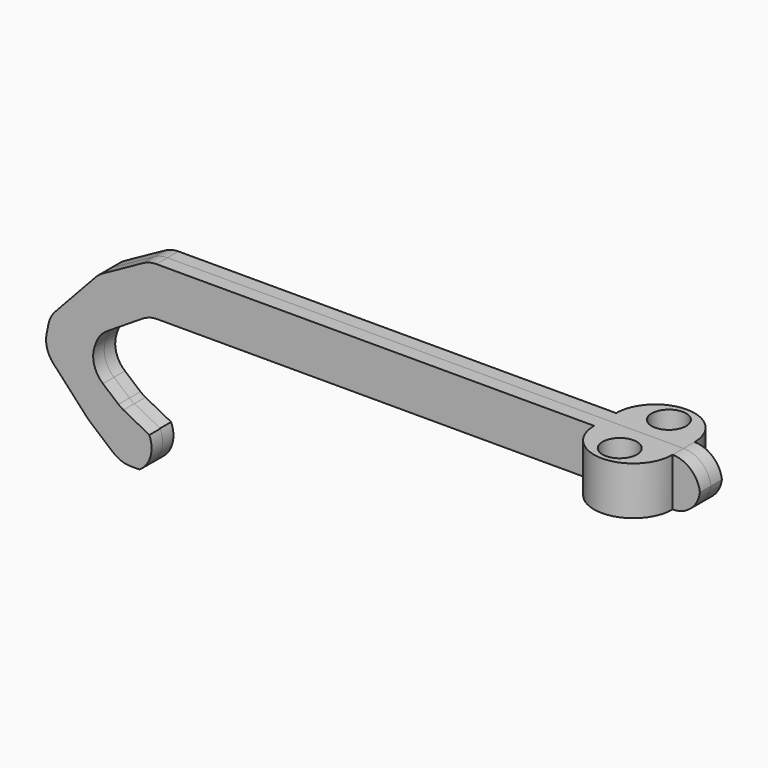
from build123d import *

# Parameters (mm, degrees)
F1_DEPTH      = 2.54
F2_T1_DEPTH   = 2.54
F2_T3_DEPTH   = 27.94
F2_T5_DEPTH   = 9.0828624111
F2_T7_DEPTH   = 6.6115491723
F2_T9_DEPTH   = 9.6489143737
F2_T11_DEPTH  = 15.5954084718
F2_T13_DEPTH  = 4.1000627259
F2_T15_DEPTH  = 11.8324981012
F4_DEPTH      = 8.89
F5_R          = 3.175
F6_DEPTH      = 25.4
F8_T1_DEPTH   = 27.7469499795
F8_2_T1_DEPTH = 27.8579477964


# Not quite as in the source:
# - a fillet or chamfer that OpenCascade refuses, or shapes differently, is made with other operations: its cross-section is extruded or revolved along the edge and cut away or added


with BuildPart() as f1:
    # F0 (on Front) → F1 (new body)
    with BuildSketch(Plane.XZ):
        Polygon((66.8724340558, 14.3756293181), (66.8724340558, 23.2656293181), (-34.7275659442, 23.2656293181), (-44.0710447729, 18.1098952889), (-53.0527345836, 8.4431990981), (-54.2040504515, 2.8466905933), (-45.9056608379, -6.1207453094), (-40.0034040213, -11.1067253005), (-36.5135949825, -11.1067253005), (-32.4798657579, -8.7494706538), (-34.7275659442, -4.9032107927), (-40.0034040213, -2.1392893977), (-45.9056608379, 2.8466905933), (-44.0710447729, 8.4431990981), (-34.7275659442, 14.3756293181), align=None)
    extrude(amount=F1_DEPTH)

    # F2: fillet of radius 5.08 on 12 edges, made by hand

    # F2_s2 → F2_t1 (join)
    with BuildSketch(Plane.XZ):
        with BuildLine():
            ThreePointArc((-33.2510846992, 14.3756293181), (-34.6688950832, 14.1737656134), (-35.9740265471, 13.5842173949))
            Line((-35.9740265471, 13.5842173949), (-34.7275659442, 14.3756293181))
            Line((-34.7275659442, 14.3756293181), (-33.2510846992, 14.3756293181))
        make_face()
        with BuildLine():
            ThreePointArc((-39.5089784479, -2.398310505), (-39.9863438705, -2.1139198711), (-40.4297931043, -1.7790937128))
            Line((-40.4297931043, -1.7790937128), (-40.0034040213, -2.1392893977))
            Line((-40.0034040213, -2.1392893977), (-39.5089784479, -2.398310505))
        make_face()
        with BuildLine():
            ThreePointArc((-43.2900772259, 0.6371548243), (-44.8991857722, 3.1320672478), (-44.8390917989, 6.1002665384))
            Line((-44.8390917989, 6.1002665384), (-45.9056608379, 2.8466905933))
            Line((-45.9056608379, 2.8466905933), (-43.2900772259, 0.6371548243))
        make_face()
        with BuildLine():
            ThreePointArc((-44.6382251268, 6.7130116573), (-43.8212350308, 8.2489469203), (-42.5339230923, 9.419159688))
            Line((-42.5339230923, 9.419159688), (-44.0710447729, 8.4431990981))
            Line((-44.0710447729, 8.4431990981), (-44.6382251268, 6.7130116573))
        make_face()
    extrude(amount=F2_T1_DEPTH)

    # F2_s4 → F2_t3 (cut)
    with BuildSketch(Plane.XZ.offset(-12.7)):
        with BuildLine():
            ThreePointArc((61.7924340558, 14.3756293181), (65.3845365042, 15.8635268697), (66.8724340558, 19.4556293181))
            Line((66.8724340558, 19.4556293181), (66.8724340558, 14.3756293181))
            Line((66.8724340558, 14.3756293181), (61.7924340558, 14.3756293181))
        make_face()
        with BuildLine():
            ThreePointArc((66.8724340558, 18.1856293181), (65.3845365042, 21.7777317665), (61.7924340558, 23.2656293181))
            Line((61.7924340558, 23.2656293181), (66.8724340558, 23.2656293181))
            Line((66.8724340558, 23.2656293181), (66.8724340558, 18.1856293181))
        make_face()
    extrude(amount=F2_T3_DEPTH, mode=Mode.SUBTRACT)

    # F2_s6 → F2_t5 (cut)
    with BuildSketch(Plane.XZ.offset(-3.2714312055)):
        with BuildLine():
            ThreePointArc((-33.418993462, 23.2656293181), (-34.6861989643, 23.1050388573), (-35.8732859172, 22.6334207413))
            Line((-35.8732859172, 22.6334207413), (-34.7275659442, 23.2656293181))
            Line((-34.7275659442, 23.2656293181), (-33.418993462, 23.2656293181))
        make_face()
    extrude(amount=F2_T5_DEPTH, mode=Mode.SUBTRACT)

    # F2_s8 → F2_t7 (cut)
    with BuildSketch(Plane.XZ.offset(-2.0357745861)):
        with BuildLine():
            ThreePointArc((-43.3580762104, 18.5033115257), (-44.0311208398, 18.0587891116), (-44.625324101, 17.513342749))
            Line((-44.625324101, 17.513342749), (-44.0710447729, 18.1098952889))
            Line((-44.0710447729, 18.1098952889), (-43.3580762104, 18.5033115257))
        make_face()
    extrude(amount=F2_T7_DEPTH, mode=Mode.SUBTRACT)

    # F2_s10 → F2_t9 (cut)
    with BuildSketch(Plane.XZ.offset(-3.5544571868)):
        with BuildLine():
            ThreePointArc((-52.0849643036, 9.4847782972), (-52.8792037753, 8.3537845313), (-53.3392248579, 7.0505793131))
            Line((-53.3392248579, 7.0505793131), (-53.0527345836, 8.4431990981))
            Line((-53.0527345836, 8.4431990981), (-52.0849643036, 9.4847782972))
        make_face()
    extrude(amount=F2_T9_DEPTH, mode=Mode.SUBTRACT)

    # F2_s12 → F2_t11 (cut)
    with BuildSketch(Plane.XZ.offset(-6.5277042359)):
        with BuildLine():
            ThreePointArc((-53.6779156077, 5.404214736), (-53.5955025606, 3.016349409), (-52.4306120015, 0.9302710989))
            Line((-52.4306120015, 0.9302710989), (-54.2040504515, 2.8466905933))
            Line((-54.2040504515, 2.8466905933), (-53.6779156077, 5.404214736))
        make_face()
    extrude(amount=F2_T11_DEPTH, mode=Mode.SUBTRACT)

    # F2_s14 → F2_t13 (cut)
    with BuildSketch(Plane.XZ.offset(-0.780031363)):
        with BuildLine():
            ThreePointArc((-46.1175787743, -5.8917417798), (-45.8990465897, -6.1138249598), (-45.6673107898, -6.3220934729))
            Line((-45.6673107898, -6.3220934729), (-45.9056608379, -6.1207453094))
            Line((-45.9056608379, -6.1207453094), (-46.1175787743, -5.8917417798))
        make_face()
    extrude(amount=F2_T13_DEPTH, mode=Mode.SUBTRACT)

    # F2_s16 → F2_t15 (cut)
    with BuildSketch(Plane.XZ.offset(-4.6462490506)):
        with BuildLine():
            ThreePointArc((-41.4231337105, -9.9073969684), (-39.890267963, -10.7974805904), (-38.144904401, -11.1067253005))
            Line((-38.144904401, -11.1067253005), (-40.0034040213, -11.1067253005))
            Line((-40.0034040213, -11.1067253005), (-41.4231337105, -9.9073969684))
        make_face()
    extrude(amount=F2_T15_DEPTH, mode=Mode.SUBTRACT)

    # F3 (on face) → F4 (join, through all)
    with BuildSketch(Plane.XY.offset(23.2656293181)):
        with BuildLine():
            Line((61.7924340558, -2.54), (47.3144340558, -2.54))
            ThreePointArc((47.3144340558, -2.54), (54.5534340558, -9.779), (61.7924340558, -2.54))
        make_face()
    extrude(amount=-F4_DEPTH)

    # F5 (on face) → F6 (cut)
    with BuildSketch(Plane.XY.offset(23.2656293181)):
        with Locations((54.5534340558, -5.6710629724)):
            Circle(F5_R)
    extrude(amount=-F6_DEPTH, mode=Mode.SUBTRACT)


with BuildPart() as f7_1:
    # F7: instance of F1
    add(f1.part.mirror(Plane.XZ))

    # F8#2: fillet of radius 5.08 on 1 edges, made by hand

    # F8_2_s2 → F8_2_t1 (cut)
    with BuildSketch(Plane.XZ.offset(-15.1989738982)):
        with BuildLine():
            ThreePointArc((-35.0346945081, -4.3776530361), (-34.4590954637, -8.0312077626), (-36.5135949825, -11.1067253005))
            Line((-36.5135949825, -11.1067253005), (-32.4798657579, -8.7494706538))
            Line((-32.4798657579, -8.7494706538), (-35.0346945081, -4.3776530361))
        make_face()
    extrude(amount=F8_2_T1_DEPTH, mode=Mode.SUBTRACT)


with BuildPart() as f1_1:
    add(f1.part)

    # F8: fillet of radius 5.08 on 1 edges, made by hand

    # F8_s2 → F8_t1 (cut)
    with BuildSketch(Plane.XZ.offset(-12.6034749897)):
        with BuildLine():
            ThreePointArc((-34.7275659442, -4.9032107927), (-34.5706782086, -8.4965419394), (-36.8325166478, -11.2930986378))
            Line((-36.8325166478, -11.2930986378), (-32.4798657579, -8.7494706538))
            Line((-32.4798657579, -8.7494706538), (-34.7275659442, -4.9032107927))
        make_face()
    extrude(amount=F8_T1_DEPTH, mode=Mode.SUBTRACT)


solid = Compound([f7_1.part, f1_1.part])
